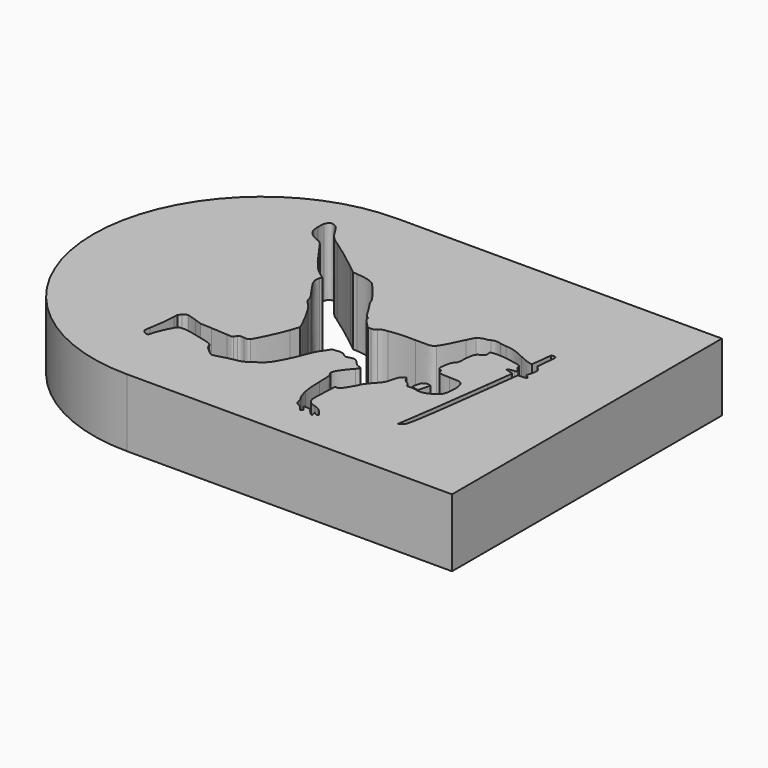
from build123d import *

# Parameters (mm, degrees)
F1_DEPTH = 5.842
F3_DEPTH = 25.4


# Not quite as in the source:
# - ends of sketch curves that miss each other by under 0.0002 mm in the source are joined


with BuildPart() as f1:
    # F0 (on Top) → F1 (new body)
    with BuildSketch(Plane.XY):
        with BuildLine():
            ThreePointArc((0, 14.5415), (-14.5415, 0), (0, -14.5415))
            Line((0, -14.5415), (28.0035, -14.5415))
            Line((28.0035, -14.5415), (28.0035, 14.5415))
            Line((28.0035, 14.5415), (0, 14.5415))
        make_face()
    extrude(amount=-F1_DEPTH)

    # F2 (on face) → F3 (cut)
    with BuildSketch(Plane.XY):
        with BuildLine():
            add(Edge.make_bspline(
                [(-3.3505654062, 10.8393135056), (-3.2275024062, 11.2703769056), (-2.9634440062, 11.3611057056), (-2.5826726062, 11.1031687056)],
                knots=[0, 0, 0, 0, 1, 1, 1, 1], degree=3))
            add(Edge.make_bspline(
                [(-3.3873192062, 10.2314661056), (-3.3936946062, 10.4726137056), (-3.3771592062, 10.7461463056), (-3.3505654062, 10.8393135056)],
                knots=[0, 0, 0, 0, 1, 1, 1, 1], degree=3))
            add(Edge.make_bspline(
                [(-2.8288748062, 9.0599165056), (-3.2257752062, 9.3249655056), (-3.3713934062, 9.6304513056), (-3.3873192062, 10.2314661056)],
                knots=[0, 0, 0, 0, 1, 1, 1, 1], degree=3))
            add(Edge.make_bspline(
                [(-2.3834096062, 8.8114283056), (-2.4746972062, 8.8454389056), (-2.6751540062, 8.9572751056), (-2.8288748062, 9.0599165056)],
                knots=[0, 0, 0, 0, 1, 1, 1, 1], degree=3))
            add(Edge.make_bspline(
                [(-1.0314946062, 7.4019823056), (-1.8672816062, 8.6240525056), (-1.8597632062, 8.6162039056), (-2.3834096062, 8.8114283056)],
                knots=[0, 0, 0, 0, 1, 1, 1, 1], degree=3))
            add(Edge.make_bspline(
                [(1.0526515938, 4.9585023056), (0.4475473938, 5.3825299056), (-0.0464826062, 5.9617261056), (-1.0314946062, 7.4019823056)],
                knots=[0, 0, 0, 0, 1, 1, 1, 1], degree=3))
            Line((1.0526515938, 4.9585023056), (1.4337023938, 4.6914975056))
            Line((1.4337023938, 4.6914975056), (1.3601947938, 4.4854019056))
            add(Edge.make_bspline(
                [(1.9874985938, 2.8520803056), (1.3599407938, 3.6886801056), (1.2126969938, 4.0720423056), (1.3601947938, 4.4854019056)],
                knots=[0, 0, 0, 0, 1, 1, 1, 1], degree=3))
            add(Edge.make_bspline(
                [(2.6965141938, 1.6528701056), (2.6965141938, 1.8108835056), (2.4284933938, 2.2641973056), (1.9874985938, 2.8520803056)],
                knots=[0, 0, 0, 0, 1, 1, 1, 1], degree=3))
            add(Edge.make_bspline(
                [(3.1149791938, 1.0430923056), (2.9105853938, 1.2135517056), (2.6965141938, 1.5254891056), (2.6965141938, 1.6528701056)],
                knots=[0, 0, 0, 0, 1, 1, 1, 1], degree=3))
            add(Edge.make_bspline(
                [(3.4769545938, 0.6155341056), (3.3687251938, 0.7749191056), (3.2058349938, 0.9673241056), (3.1149791938, 1.0430923056)],
                knots=[0, 0, 0, 0, 1, 1, 1, 1], degree=3))
            add(Edge.make_bspline(
                [(4.6368709938, -1.5235268944), (4.4779685938, -1.1114626944), (3.7972231938, 0.1439069056), (3.4769545938, 0.6155341056)],
                knots=[0, 0, 0, 0, 1, 1, 1, 1], degree=3))
            Line((4.6368709938, -1.5235268944), (4.7843433938, -1.9058984944))
            Line((4.7843433938, -1.9058984944), (4.5295305938, -2.6590846944))
            add(Edge.make_bspline(
                [(3.2766247938, -5.3463792944), (3.5066725938, -5.0567938944), (4.2781721938, -3.4020600944), (4.5295305938, -2.6590846944)],
                knots=[0, 0, 0, 0, 1, 1, 1, 1], degree=3))
            add(Edge.make_bspline(
                [(2.8130493938, -5.4498080944), (3.1617659938, -5.4824724944), (3.1699701938, -5.4806436944), (3.2766247938, -5.3463792944)],
                knots=[0, 0, 0, 0, 1, 1, 1, 1], degree=3))
            add(Edge.make_bspline(
                [(2.3198829938, -5.5551926944), (2.4545029938, -5.4200900944), (2.4671521938, -5.4173976944), (2.8130493938, -5.4498080944)],
                knots=[0, 0, 0, 0, 1, 1, 1, 1], degree=3))
            add(Edge.make_bspline(
                [(2.1355297938, -5.7769092944), (2.1609297938, -5.7312146944), (2.2438861938, -5.6314434944), (2.3198829938, -5.5551926944)],
                knots=[0, 0, 0, 0, 1, 1, 1, 1], degree=3))
            add(Edge.make_bspline(
                [(1.6304253938, -5.8127232944), (2.0435309938, -5.8552428944), (2.0939753938, -5.8516614944), (2.1355297938, -5.7769092944)],
                knots=[0, 0, 0, 0, 1, 1, 1, 1], degree=3))
            add(Edge.make_bspline(
                [(0.2032247938, -5.7259568944), (0.7357865938, -5.7476992944), (1.3780255938, -5.7867136944), (1.6304253938, -5.8127232944)],
                knots=[0, 0, 0, 0, 1, 1, 1, 1], degree=3))
            Line((0.2032247938, -5.7259568944), (-0.7650486062, -5.6864598944))
            Line((-0.7650486062, -5.6864598944), (-1.3459974062, -5.4790942944))
            add(Edge.make_bspline(
                [(-2.1341086062, -5.2478526944), (-2.0201642062, -5.2609844944), (-1.6655294062, -5.3650482944), (-1.3459974062, -5.4790942944)],
                knots=[0, 0, 0, 0, 1, 1, 1, 1], degree=3))
            add(Edge.make_bspline(
                [(-2.5577298062, -5.4404354944), (-2.3551648062, -5.2378704944), (-2.3279106062, -5.2254752944), (-2.1341086062, -5.2478526944)],
                knots=[0, 0, 0, 0, 1, 1, 1, 1], degree=3))
            Line((-2.5577298062, -5.4404354944), (-2.7741886062, -5.6568942944))
            Line((-2.7741886062, -5.6568942944), (-2.7741886062, -6.0245084944))
            add(Edge.make_bspline(
                [(-3.0388058062, -8.2597592944), (-2.9170128062, -7.6244290944), (-2.7741886062, -6.4181576944), (-2.7741886062, -6.0245084944)],
                knots=[0, 0, 0, 0, 1, 1, 1, 1], degree=3))
            add(Edge.make_bspline(
                [(-2.9799540062, -8.9563288944), (-3.1350210062, -8.7916860944), (-3.1367990062, -8.7707818944), (-3.0388058062, -8.2597592944)],
                knots=[0, 0, 0, 0, 1, 1, 1, 1], degree=3))
            add(Edge.make_bspline(
                [(-2.5392640062, -9.1113958944), (-2.6438866062, -9.1760642944), (-2.8369520062, -9.1081446944), (-2.9799540062, -8.9563288944)],
                knots=[0, 0, 0, 0, 1, 1, 1, 1], degree=3))
            add(Edge.make_bspline(
                [(-2.4057108062, -8.7382190944), (-2.4435822062, -8.9214800944), (-2.5037040062, -9.0894248944), (-2.5392640062, -9.1113958944)],
                knots=[0, 0, 0, 0, 1, 1, 1, 1], degree=3))
            add(Edge.make_bspline(
                [(-1.6354304062, -7.0924006944), (-1.8189708062, -7.2759156944), (-2.3284694062, -8.3645342944), (-2.4057108062, -8.7382190944)],
                knots=[0, 0, 0, 0, 1, 1, 1, 1], degree=3))
            add(Edge.make_bspline(
                [(-1.2150604062, -6.9773132944), (-1.4721846062, -6.9768306944), (-1.5379198062, -6.9948900944), (-1.6354304062, -7.0924006944)],
                knots=[0, 0, 0, 0, 1, 1, 1, 1], degree=3))
            add(Edge.make_bspline(
                [(0.8847829938, -7.3951940944), (-0.0074682062, -7.1444198944), (-0.8440934062, -6.9779228944), (-1.2150604062, -6.9773132944)],
                knots=[0, 0, 0, 0, 1, 1, 1, 1], degree=3))
            add(Edge.make_bspline(
                [(1.6190461938, -7.7483556944), (1.5512535938, -7.5863544944), (1.5318733938, -7.5770326944), (0.8847829938, -7.3951940944)],
                knots=[0, 0, 0, 0, 1, 1, 1, 1], degree=3))
            add(Edge.make_bspline(
                [(1.8173947938, -8.0838388944), (1.7466049938, -7.9908240944), (1.6573493938, -7.8398464944), (1.6190461938, -7.7483556944)],
                knots=[0, 0, 0, 0, 1, 1, 1, 1], degree=3))
            add(Edge.make_bspline(
                [(2.6697171938, -8.7680894944), (2.5522929938, -8.7680894944), (2.0018495938, -8.3261802944), (1.8173947938, -8.0838388944)],
                knots=[0, 0, 0, 0, 1, 1, 1, 1], degree=3))
            add(Edge.make_bspline(
                [(3.4470079938, -8.5743636944), (3.0742629938, -8.6809166944), (2.7244795938, -8.7680894944), (2.6697171938, -8.7680894944)],
                knots=[0, 0, 0, 0, 1, 1, 1, 1], degree=3))
            add(Edge.make_bspline(
                [(4.4755301938, -8.3370006944), (4.2825663938, -8.3610036944), (3.8197529938, -8.4678106944), (3.4470079938, -8.5743636944)],
                knots=[0, 0, 0, 0, 1, 1, 1, 1], degree=3))
            add(Edge.make_bspline(
                [(5.7562235938, -7.6816552944), (4.9934869938, -8.2261550944), (4.8735227938, -8.2875214944), (4.4755301938, -8.3370006944)],
                knots=[0, 0, 0, 0, 1, 1, 1, 1], degree=3))
            add(Edge.make_bspline(
                [(6.4918837938, -6.9844506944), (6.3146425938, -7.2510744944), (6.1780667938, -7.3805128944), (5.7562235938, -7.6816552944)],
                knots=[0, 0, 0, 0, 1, 1, 1, 1], degree=3))
            add(Edge.make_bspline(
                [(7.4134719938, -5.1370832944), (7.1996801938, -5.7229342944), (6.8062849938, -6.5115534944), (6.4918837938, -6.9844506944)],
                knots=[0, 0, 0, 0, 1, 1, 1, 1], degree=3))
            add(Edge.make_bspline(
                [(8.0773009938, -3.7124480944), (7.9343497938, -3.8755160944), (7.6553561938, -4.4742702944), (7.4134719938, -5.1370832944)],
                knots=[0, 0, 0, 0, 1, 1, 1, 1], degree=3))
            add(Edge.make_bspline(
                [(8.3400131938, -3.3308892944), (8.2583013938, -3.4691414944), (8.1400897938, -3.6408454944), (8.0773009938, -3.7124480944)],
                knots=[0, 0, 0, 0, 1, 1, 1, 1], degree=3))
            add(Edge.make_bspline(
                [(8.6434923938, -3.0716060944), (8.5114377938, -3.0783624944), (8.4666321938, -3.1166148944), (8.3400131938, -3.3308892944)],
                knots=[0, 0, 0, 0, 1, 1, 1, 1], degree=3))
            add(Edge.make_bspline(
                [(8.9918025938, -3.0366302944), (8.8854527938, -3.0514892944), (8.7287093938, -3.0672372944), (8.6434923938, -3.0716060944)],
                knots=[0, 0, 0, 0, 1, 1, 1, 1], degree=3))
            add(Edge.make_bspline(
                [(9.6258627938, -3.2060990944), (9.4464371938, -3.0459012944), (9.2674433938, -2.9980730944), (8.9918025938, -3.0366302944)],
                knots=[0, 0, 0, 0, 1, 1, 1, 1], degree=3))
            add(Edge.make_bspline(
                [(10.2087927938, -3.2670082944), (9.8359461938, -3.3716308944), (9.8079807938, -3.3686844944), (9.6258627938, -3.2060990944)],
                knots=[0, 0, 0, 0, 1, 1, 1, 1], degree=3))
            add(Edge.make_bspline(
                [(11.0254027938, -3.5898930944), (10.7011463938, -3.2156240944), (10.5728001938, -3.1648748944), (10.2087927938, -3.2670082944)],
                knots=[0, 0, 0, 0, 1, 1, 1, 1], degree=3))
            add(Edge.make_bspline(
                [(11.4640099938, -3.9033290944), (11.3044725938, -3.8763796944), (11.2233957938, -3.8184422944), (11.0254027938, -3.5898930944)],
                knots=[0, 0, 0, 0, 1, 1, 1, 1], degree=3))
            add(Edge.make_bspline(
                [(11.6861837938, -4.0052846944), (11.6716549938, -3.9674132944), (11.5716805938, -3.9215154944), (11.4640099938, -3.9033290944)],
                knots=[0, 0, 0, 0, 1, 1, 1, 1], degree=3))
            add(Edge.make_bspline(
                [(11.5012717938, -4.3054872944), (11.6230139938, -4.1722642944), (11.7014237938, -4.0449848944), (11.6861837938, -4.0052846944)],
                knots=[0, 0, 0, 0, 1, 1, 1, 1], degree=3))
            add(Edge.make_bspline(
                [(10.5397801938, -5.7960100944), (10.5412533938, -5.5009890944), (10.8591089938, -5.0082290944), (11.5012717938, -4.3054872944)],
                knots=[0, 0, 0, 0, 1, 1, 1, 1], degree=3))
            add(Edge.make_bspline(
                [(10.6534959938, -6.0177774944), (10.5908087938, -5.9253722944), (10.5396277938, -5.8256010944), (10.5397801938, -5.7960100944)],
                knots=[0, 0, 0, 0, 1, 1, 1, 1], degree=3))
            add(Edge.make_bspline(
                [(10.7944913938, -7.3195782944), (10.7685833938, -6.2311374944), (10.7629445938, -6.1790420944), (10.6534959938, -6.0177774944)],
                knots=[0, 0, 0, 0, 1, 1, 1, 1], degree=3))
            add(Edge.make_bspline(
                [(10.9251997938, -8.9564812944), (10.8437673938, -8.5615874944), (10.8156749938, -8.2095942944), (10.7944913938, -7.3195782944)],
                knots=[0, 0, 0, 0, 1, 1, 1, 1], degree=3))
            add(Edge.make_bspline(
                [(11.3379243938, -10.0268626944), (11.1851433938, -9.8455066944), (11.0204243938, -9.4182786944), (10.9251997938, -8.9564812944)],
                knots=[0, 0, 0, 0, 1, 1, 1, 1], degree=3))
            add(Edge.make_bspline(
                [(11.4311169938, -10.3223408944), (11.4135147938, -10.1997604944), (11.3715539938, -10.0667914944), (11.3379243938, -10.0268626944)],
                knots=[0, 0, 0, 0, 1, 1, 1, 1], degree=3))
            add(Edge.make_bspline(
                [(11.8227087938, -10.8226446944), (11.5826025938, -10.7223400944), (11.4674643938, -10.5752486944), (11.4311169938, -10.3223408944)],
                knots=[0, 0, 0, 0, 1, 1, 1, 1], degree=3))
            add(Edge.make_bspline(
                [(12.1231907938, -11.0862966944), (12.0489465938, -10.9793118944), (11.9137169938, -10.8606938944), (11.8227087938, -10.8226446944)],
                knots=[0, 0, 0, 0, 1, 1, 1, 1], degree=3))
            add(Edge.make_bspline(
                [(12.4579627938, -11.2805050944), (12.3635509938, -11.3588640944), (12.2779021938, -11.3092070944), (12.1231907938, -11.0862966944)],
                knots=[0, 0, 0, 0, 1, 1, 1, 1], degree=3))
            add(Edge.make_bspline(
                [(12.3512319938, -10.9554104944), (12.5451863938, -11.1820038944), (12.5519173938, -11.2025270944), (12.4579627938, -11.2805050944)],
                knots=[0, 0, 0, 0, 1, 1, 1, 1], degree=3))
            Line((12.3512319938, -10.9554104944), (12.1780039938, -10.7530486944))
            Line((12.1780039938, -10.7530486944), (12.4270255938, -10.7530486944))
            add(Edge.make_bspline(
                [(12.9128767938, -10.9738508944), (12.8514849938, -10.8123576944), (12.7209543938, -10.7530486944), (12.4270255938, -10.7530486944)],
                knots=[0, 0, 0, 0, 1, 1, 1, 1], degree=3))
            add(Edge.make_bspline(
                [(13.0289547938, -11.0919354944), (12.9898133938, -11.0919354944), (12.9375655938, -11.0387986944), (12.9128767938, -10.9738508944)],
                knots=[0, 0, 0, 0, 1, 1, 1, 1], degree=3))
            add(Edge.make_bspline(
                [(13.1637271938, -11.2250822944), (13.1287513938, -11.1518540944), (13.0680961938, -11.0919354944), (13.0289547938, -11.0919354944)],
                knots=[0, 0, 0, 0, 1, 1, 1, 1], degree=3))
            add(Edge.make_bspline(
                [(13.4267187938, -11.3095626944), (13.4825225938, -11.4550284944), (13.2357107938, -11.3757296944), (13.1637271938, -11.2250822944)],
                knots=[0, 0, 0, 0, 1, 1, 1, 1], degree=3))
            add(Edge.make_bspline(
                [(13.3651999938, -11.0995554944), (13.3818369938, -11.1702944944), (13.4095229938, -11.2648078944), (13.4267187938, -11.3095626944)],
                knots=[0, 0, 0, 0, 1, 1, 1, 1], degree=3))
            Line((13.3651999938, -11.0995554944), (13.3348977938, -10.9709044944))
            Line((13.3348977938, -10.9709044944), (13.4399013938, -11.0798450944))
            add(Edge.make_bspline(
                [(13.7656817938, -11.1161162944), (13.8107159938, -11.2334642944), (13.5611863938, -11.2056766944), (13.4399013938, -11.0798450944)],
                knots=[0, 0, 0, 0, 1, 1, 1, 1], degree=3))
            add(Edge.make_bspline(
                [(13.2264397938, -10.4739026944), (13.4143489938, -10.6175650944), (13.7090397938, -10.9685422944), (13.7656817938, -11.1161162944)],
                knots=[0, 0, 0, 0, 1, 1, 1, 1], degree=3))
            add(Edge.make_bspline(
                [(12.7633723938, -10.2558944944), (12.9115559938, -10.2943754944), (13.1199375938, -10.3924702944), (13.2264397938, -10.4739026944)],
                knots=[0, 0, 0, 0, 1, 1, 1, 1], degree=3))
            add(Edge.make_bspline(
                [(12.0906279938, -9.8329336944), (12.2213871938, -10.0686202944), (12.3476251938, -10.1479698944), (12.7633723938, -10.2558944944)],
                knots=[0, 0, 0, 0, 1, 1, 1, 1], degree=3))
            add(Edge.make_bspline(
                [(12.0199905938, -8.0903158944), (11.9475751938, -9.4684690944), (11.9522487938, -9.5834802944), (12.0906279938, -9.8329336944)],
                knots=[0, 0, 0, 0, 1, 1, 1, 1], degree=3))
            Line((12.0199905938, -8.0903158944), (12.0645167938, -7.2430734944))
            Line((12.0645167938, -7.2430734944), (12.2447551938, -7.2281382944))
            add(Edge.make_bspline(
                [(12.5261109938, -7.0829010944), (12.4546353938, -7.1749760944), (12.3720853938, -7.2175972944), (12.2447551938, -7.2281382944)],
                knots=[0, 0, 0, 0, 1, 1, 1, 1], degree=3))
            add(Edge.make_bspline(
                [(13.1625333938, -6.0085572944), (13.1052055938, -6.1597126944), (12.6621025938, -6.9077426944), (12.5261109938, -7.0829010944)],
                knots=[0, 0, 0, 0, 1, 1, 1, 1], degree=3))
            add(Edge.make_bspline(
                [(13.8604237938, -5.0402838944), (13.5216131938, -5.3899402944), (13.2589009938, -5.7544302944), (13.1625333938, -6.0085572944)],
                knots=[0, 0, 0, 0, 1, 1, 1, 1], degree=3))
            add(Edge.make_bspline(
                [(14.4640547938, -3.8166642944), (14.3186397938, -4.4798836944), (14.2306795938, -4.6581916944), (13.8604237938, -5.0402838944)],
                knots=[0, 0, 0, 0, 1, 1, 1, 1], degree=3))
            add(Edge.make_bspline(
                [(14.7380445938, -3.3410492944), (14.5629115938, -3.5024916944), (14.5145245938, -3.5864894944), (14.4640547938, -3.8166642944)],
                knots=[0, 0, 0, 0, 1, 1, 1, 1], degree=3))
            add(Edge.make_bspline(
                [(15.0205687938, -3.2028986944), (14.9639267938, -3.1559086944), (14.9106121938, -3.1819690944), (14.7380445938, -3.3410492944)],
                knots=[0, 0, 0, 0, 1, 1, 1, 1], degree=3))
            add(Edge.make_bspline(
                [(15.0903679938, -3.3467134944), (15.0903679938, -3.2994948944), (15.0589481938, -3.2347756944), (15.0205687938, -3.2028986944)],
                knots=[0, 0, 0, 0, 1, 1, 1, 1], degree=3))
            add(Edge.make_bspline(
                [(15.5182309938, -3.7548406944), (15.3689043938, -3.7074442944), (15.0903679938, -3.4417602944), (15.0903679938, -3.3467134944)],
                knots=[0, 0, 0, 0, 1, 1, 1, 1], degree=3))
            add(Edge.make_bspline(
                [(15.6937449938, -3.9540528944), (15.6496505938, -3.8611142944), (15.5706565938, -3.7714776944), (15.5182309938, -3.7548406944)],
                knots=[0, 0, 0, 0, 1, 1, 1, 1], degree=3))
            add(Edge.make_bspline(
                [(16.0009833938, -4.0939052944), (15.7787333938, -4.1223786944), (15.7722055938, -4.1194068944), (15.6937449938, -3.9540528944)],
                knots=[0, 0, 0, 0, 1, 1, 1, 1], degree=3))
            add(Edge.make_bspline(
                [(16.5166287938, -4.1410222944), (16.3357553938, -4.0932448944), (16.1433249938, -4.0756680944), (16.0009833938, -4.0939052944)],
                knots=[0, 0, 0, 0, 1, 1, 1, 1], degree=3))
            add(Edge.make_bspline(
                [(17.4719227938, -4.1167652944), (17.1669449938, -4.2369834944), (16.9049947938, -4.2436382944), (16.5166287938, -4.1410222944)],
                knots=[0, 0, 0, 0, 1, 1, 1, 1], degree=3))
            add(Edge.make_bspline(
                [(18.3957715938, -3.4327940944), (18.3063127938, -3.6234972944), (17.8314343938, -3.9750586944), (17.4719227938, -4.1167652944)],
                knots=[0, 0, 0, 0, 1, 1, 1, 1], degree=3))
            add(Edge.make_bspline(
                [(18.5272673938, -2.0712016944), (18.5881511938, -2.4226868944), (18.5151769938, -3.1782606944), (18.3957715938, -3.4327940944)],
                knots=[0, 0, 0, 0, 1, 1, 1, 1], degree=3))
            add(Edge.make_bspline(
                [(17.2386745938, -1.3329252944), (18.3122055938, -1.3384116944), (18.4100463938, -1.3944694944), (18.5272673938, -2.0712016944)],
                knots=[0, 0, 0, 0, 1, 1, 1, 1], degree=3))
            add(Edge.make_bspline(
                [(16.1944805938, -1.0538554944), (16.2170103938, -1.2854018944), (16.3783765938, -1.3285310944), (17.2386745938, -1.3329252944)],
                knots=[0, 0, 0, 0, 1, 1, 1, 1], degree=3))
            add(Edge.make_bspline(
                [(16.0527231938, -0.8410796944), (16.1431725938, -0.8842088944), (16.1839141938, -0.9453974944), (16.1944805938, -1.0538554944)],
                knots=[0, 0, 0, 0, 1, 1, 1, 1], degree=3))
            add(Edge.make_bspline(
                [(15.8627565938, -0.2858864944), (15.8029903938, -0.6743286944), (15.8224975938, -0.7313008944), (16.0527231938, -0.8410796944)],
                knots=[0, 0, 0, 0, 1, 1, 1, 1], degree=3))
            add(Edge.make_bspline(
                [(16.1682931938, 0.6071267056), (16.0011357938, 0.4167283056), (15.9461701938, 0.2560225056), (15.8627565938, -0.2858864944)],
                knots=[0, 0, 0, 0, 1, 1, 1, 1], degree=3))
            add(Edge.make_bspline(
                [(16.3486839938, 1.3932059056), (16.3227251938, 0.7919879056), (16.3199311938, 0.7797959056), (16.1682931938, 0.6071267056)],
                knots=[0, 0, 0, 0, 1, 1, 1, 1], degree=3))
            add(Edge.make_bspline(
                [(16.7442127938, 2.5041003056), (16.4755569938, 2.3565263056), (16.3785035938, 2.0839335056), (16.3486839938, 1.3932059056)],
                knots=[0, 0, 0, 0, 1, 1, 1, 1], degree=3))
            add(Edge.make_bspline(
                [(17.0992285938, 2.9984605056), (17.1337725938, 2.7473053056), (17.0991015938, 2.6990199056), (16.7442127938, 2.5041003056)],
                knots=[0, 0, 0, 0, 1, 1, 1, 1], degree=3))
            Line((17.0992285938, 2.9984605056), (17.0674023938, 3.2298545056))
            Line((17.0674023938, 3.2298545056), (17.3890425938, 3.2642969056))
            add(Edge.make_bspline(
                [(18.9392299938, 3.1356967056), (18.2177429938, 3.2684117056), (17.7724047938, 3.3053687056), (17.3890425938, 3.2642969056)],
                knots=[0, 0, 0, 0, 1, 1, 1, 1], degree=3))
            add(Edge.make_bspline(
                [(19.8777091938, 2.7538585056), (19.8109833938, 2.9765149056), (19.8163681938, 2.9743305056), (18.9392299938, 3.1356967056)],
                knots=[0, 0, 0, 0, 1, 1, 1, 1], degree=3))
            add(Edge.make_bspline(
                [(20.0791311938, 2.3960995056), (20.0004419938, 2.4857107056), (19.9098147938, 2.6466959056), (19.8777091938, 2.7538585056)],
                knots=[0, 0, 0, 0, 1, 1, 1, 1], degree=3))
            add(Edge.make_bspline(
                [(20.0406247938, 2.1246243056), (20.2599537938, 2.1249545056), (20.2679039938, 2.1810885056), (20.0791311938, 2.3960995056)],
                knots=[0, 0, 0, 0, 1, 1, 1, 1], degree=3))
            add(Edge.make_bspline(
                [(19.4959979938, 1.9811397056), (19.4959979938, 2.0391533056), (19.8192129938, 2.1242941056), (20.0406247938, 2.1246243056)],
                knots=[0, 0, 0, 0, 1, 1, 1, 1], degree=3))
            add(Edge.make_bspline(
                [(19.9959969938, 1.8113915056), (19.7177907938, 1.8582037056), (19.4959979938, 1.9335147056), (19.4959979938, 1.9811397056)],
                knots=[0, 0, 0, 0, 1, 1, 1, 1], degree=3))
            add(Edge.make_bspline(
                [(20.1535023938, 1.6015621056), (20.1808581938, 1.7774063056), (20.1783943938, 1.7807083056), (19.9959969938, 1.8113915056)],
                knots=[0, 0, 0, 0, 1, 1, 1, 1], degree=3))
            add(Edge.make_bspline(
                [(19.8809095938, -0.5378290944), (20.0155549938, 0.5405787056), (20.1382115938, 1.5032895056), (20.1535023938, 1.6015621056)],
                knots=[0, 0, 0, 0, 1, 1, 1, 1], degree=3))
            add(Edge.make_bspline(
                [(18.7495427938, -8.7318690944), (18.8561211938, -8.2594798944), (19.4904861938, -3.6651024944), (19.8809095938, -0.5378290944)],
                knots=[0, 0, 0, 0, 1, 1, 1, 1], degree=3))
            add(Edge.make_bspline(
                [(18.9989199938, -8.6381176944), (18.7602361938, -8.8145968944), (18.7281559938, -8.8266618944), (18.7495427938, -8.7318690944)],
                knots=[0, 0, 0, 0, 1, 1, 1, 1], degree=3))
            add(Edge.make_bspline(
                [(19.2281549938, -8.2700462944), (19.1763135938, -8.4499798944), (19.1105529938, -8.5555676944), (18.9989199938, -8.6381176944)],
                knots=[0, 0, 0, 0, 1, 1, 1, 1], degree=3))
            add(Edge.make_bspline(
                [(20.2715869938, -1.0703908944), (19.8048365938, -4.8771904944), (19.3990969938, -7.6768038944), (19.2281549938, -8.2700462944)],
                knots=[0, 0, 0, 0, 1, 1, 1, 1], degree=3))
            add(Edge.make_bspline(
                [(20.5965799938, 1.5197233056), (20.5761837938, 1.3866019056), (20.4299305938, 0.2210467056), (20.2715869938, -1.0703908944)],
                knots=[0, 0, 0, 0, 1, 1, 1, 1], degree=3))
            Line((20.5965799938, 1.5197233056), (20.6336893938, 1.7618107056))
            Line((20.6336893938, 1.7618107056), (20.9483953938, 1.7860169056))
            add(Edge.make_bspline(
                [(21.3071449938, 1.9844671056), (21.4210385938, 1.8586355056), (21.3448893938, 1.8164969056), (20.9483953938, 1.7860169056)],
                knots=[0, 0, 0, 0, 1, 1, 1, 1], degree=3))
            add(Edge.make_bspline(
                [(21.1616029938, 2.0764913056), (21.1958421938, 2.0764913056), (21.2613487938, 2.0350893056), (21.3071449938, 1.9844671056)],
                knots=[0, 0, 0, 0, 1, 1, 1, 1], degree=3))
            add(Edge.make_bspline(
                [(21.1414861938, 2.4460613056), (21.0450677938, 2.1578729056), (21.0494873938, 2.0764913056), (21.1616029938, 2.0764913056)],
                knots=[0, 0, 0, 0, 1, 1, 1, 1], degree=3))
            add(Edge.make_bspline(
                [(21.2376759938, 2.9657199056), (21.2370409938, 2.8361291056), (21.1937339938, 2.6022713056), (21.1414861938, 2.4460613056)],
                knots=[0, 0, 0, 0, 1, 1, 1, 1], degree=3))
            add(Edge.make_bspline(
                [(21.0402163938, 3.4000345056), (21.2190069938, 3.2212693056), (21.2387427938, 3.1778099056), (21.2376759938, 2.9657199056)],
                knots=[0, 0, 0, 0, 1, 1, 1, 1], degree=3))
            Line((21.0402163938, 3.4000345056), (20.8415629938, 3.5987133056))
            Line((20.8415629938, 3.5987133056), (20.9271863938, 4.4521025056))
            add(Edge.make_bspline(
                [(20.9821265938, 5.3854509056), (20.9989921938, 5.3414581056), (20.9742779938, 4.9214437056), (20.9271863938, 4.4521025056)],
                knots=[0, 0, 0, 0, 1, 1, 1, 1], degree=3))
            add(Edge.make_bspline(
                [(20.5589879938, 5.4049073056), (20.5623153938, 5.5011987056), (20.9444329938, 5.4836473056), (20.9821265938, 5.3854509056)],
                knots=[0, 0, 0, 0, 1, 1, 1, 1], degree=3))
            add(Edge.make_bspline(
                [(20.3552545938, 3.6458303056), (20.3779367938, 3.6684871056), (20.5503773938, 5.1575367056), (20.5589879938, 5.4049073056)],
                knots=[0, 0, 0, 0, 1, 1, 1, 1], degree=3))
            add(Edge.make_bspline(
                [(19.1252595938, 4.0586057056), (19.7361549938, 3.7568283056), (20.2828137938, 3.5733895056), (20.3552545938, 3.6458303056)],
                knots=[0, 0, 0, 0, 1, 1, 1, 1], degree=3))
            add(Edge.make_bspline(
                [(17.3686717938, 4.5945711056), (17.8184041938, 4.5936059056), (18.4037471938, 4.4149931056), (19.1252595938, 4.0586057056)],
                knots=[0, 0, 0, 0, 1, 1, 1, 1], degree=3))
            add(Edge.make_bspline(
                [(16.8332397938, 4.6666055056), (16.9796961938, 4.6273117056), (17.2206405938, 4.5948759056), (17.3686717938, 4.5945711056)],
                knots=[0, 0, 0, 0, 1, 1, 1, 1], degree=3))
            add(Edge.make_bspline(
                [(16.0228527938, 4.6423993056), (16.2370001938, 4.7571565056), (16.4699435938, 4.7641161056), (16.8332397938, 4.6666055056)],
                knots=[0, 0, 0, 0, 1, 1, 1, 1], degree=3))
            add(Edge.make_bspline(
                [(15.7413445938, 4.5455745056), (15.7968181938, 4.5455745056), (15.9235133938, 4.5891609056), (16.0228527938, 4.6423993056)],
                knots=[0, 0, 0, 0, 1, 1, 1, 1], degree=3))
            add(Edge.make_bspline(
                [(15.0342339938, 4.2683335056), (15.1544013938, 4.3975941056), (15.5318453938, 4.5455745056), (15.7413445938, 4.5455745056)],
                knots=[0, 0, 0, 0, 1, 1, 1, 1], degree=3))
            add(Edge.make_bspline(
                [(14.6797769938, 3.6257135056), (14.8060657938, 3.9053167056), (14.9655777938, 4.1944957056), (15.0342339938, 4.2683335056)],
                knots=[0, 0, 0, 0, 1, 1, 1, 1], degree=3))
            add(Edge.make_bspline(
                [(13.6749275938, 1.7227709056), (13.8424913938, 1.9181985056), (14.2989039938, 2.7825605056), (14.6797769938, 3.6257135056)],
                knots=[0, 0, 0, 0, 1, 1, 1, 1], degree=3))
            add(Edge.make_bspline(
                [(12.0403105938, 1.4744351056), (13.3081769938, 1.4404245056), (13.4515091938, 1.4621923056), (13.6749275938, 1.7227709056)],
                knots=[0, 0, 0, 0, 1, 1, 1, 1], degree=3))
            add(Edge.make_bspline(
                [(9.7890831938, 1.3514229056), (10.7314993938, 1.4874653056), (11.0025427938, 1.5022735056), (12.0403105938, 1.4744351056)],
                knots=[0, 0, 0, 0, 1, 1, 1, 1], degree=3))
            add(Edge.make_bspline(
                [(9.0654371938, 1.0833259056), (9.2479615938, 1.2658503056), (9.2808799938, 1.2780423056), (9.7890831938, 1.3514229056)],
                knots=[0, 0, 0, 0, 1, 1, 1, 1], degree=3))
            add(Edge.make_bspline(
                [(8.6398093938, 0.9145683056), (8.8686125938, 0.9145683056), (8.9150945938, 0.9330087056), (9.0654371938, 1.0833259056)],
                knots=[0, 0, 0, 0, 1, 1, 1, 1], degree=3))
            Line((8.6398093938, 0.9145683056), (8.3829645938, 0.9145683056))
            Line((8.3829645938, 0.9145683056), (7.9878675938, 1.3139833056))
            add(Edge.make_bspline(
                [(7.5774289938, 1.8586355056), (7.5886557938, 1.7523365056), (7.6987139938, 1.6062865056), (7.9878675938, 1.3139833056)],
                knots=[0, 0, 0, 0, 1, 1, 1, 1], degree=3))
            add(Edge.make_bspline(
                [(7.4155039938, 2.0746879056), (7.5224125938, 2.0230243056), (7.5662275938, 1.9645789056), (7.5774289938, 1.8586355056)],
                knots=[0, 0, 0, 0, 1, 1, 1, 1], degree=3))
            add(Edge.make_bspline(
                [(6.9910191938, 2.6421493056), (7.1940413938, 2.2793357056), (7.3084175938, 2.1264277056), (7.4155039938, 2.0746879056)],
                knots=[0, 0, 0, 0, 1, 1, 1, 1], degree=3))
            add(Edge.make_bspline(
                [(6.4762627938, 3.4516727056), (6.6065139938, 3.2795623056), (6.8381619938, 2.9153009056), (6.9910191938, 2.6421493056)],
                knots=[0, 0, 0, 0, 1, 1, 1, 1], degree=3))
            add(Edge.make_bspline(
                [(6.1641729938, 4.0219281056), (6.2072259938, 3.8747097056), (6.3408045938, 3.6306411056), (6.4762627938, 3.4516727056)],
                knots=[0, 0, 0, 0, 1, 1, 1, 1], degree=3))
            add(Edge.make_bspline(
                [(5.4283857938, 5.1023425056), (5.9508129938, 4.4513913056), (6.1046607938, 4.2254837056), (6.1641729938, 4.0219281056)],
                knots=[0, 0, 0, 0, 1, 1, 1, 1], degree=3))
            add(Edge.make_bspline(
                [(4.6431193938, 6.0583477056), (4.7117247938, 5.9852211056), (5.0651149938, 5.5549959056), (5.4283857938, 5.1023425056)],
                knots=[0, 0, 0, 0, 1, 1, 1, 1], degree=3))
            add(Edge.make_bspline(
                [(2.9330643938, 6.5501933056), (3.6955215938, 6.5021365056), (4.4232061938, 6.2928405056), (4.6431193938, 6.0583477056)],
                knots=[0, 0, 0, 0, 1, 1, 1, 1], degree=3))
            Line((2.9330643938, 6.5501933056), (2.5853891938, 6.5721135056))
            Line((2.5853891938, 6.5721135056), (1.9268687938, 7.1002303056))
            add(Edge.make_bspline(
                [(-0.8054600062, 9.1349227056), (-0.0911866062, 8.6574789056), (0.9765277938, 7.8623827056), (1.9268687938, 7.1002303056)],
                knots=[0, 0, 0, 0, 1, 1, 1, 1], degree=3))
            add(Edge.make_bspline(
                [(-2.0946624062, 10.4762205056), (-1.7152372062, 9.8135345056), (-1.5257278062, 9.6163797056), (-0.8054600062, 9.1349227056)],
                knots=[0, 0, 0, 0, 1, 1, 1, 1], degree=3))
            add(Edge.make_bspline(
                [(-2.5826726062, 11.1031687056), (-2.4230082062, 10.9950155056), (-2.3045934062, 10.8428949056), (-2.0946624062, 10.4762205056)],
                knots=[0, 0, 0, 0, 1, 1, 1, 1], degree=3))
        make_face()
        with BuildLine():
            add(Edge.make_bspline(
                [(16.1483795938, -3.9169942944), (16.1933629938, -3.9879110944), (16.6773853938, -4.1289318944), (16.7068239938, -4.0797066944)],
                knots=[0, 0, 0, 0, 1, 1, 1, 1], degree=3))
            add(Edge.make_bspline(
                [(16.1126417938, -3.8299484944), (16.1103811938, -3.8432580944), (16.1264593938, -3.8824248944), (16.1483795938, -3.9169942944)],
                knots=[0, 0, 0, 0, 1, 1, 1, 1], degree=3))
            add(Edge.make_bspline(
                [(16.2792657938, -3.1739426944), (16.2174929938, -3.3865152944), (16.1285167938, -3.7367812944), (16.1126417938, -3.8299484944)],
                knots=[0, 0, 0, 0, 1, 1, 1, 1], degree=3))
            Line((16.2792657938, -3.1739426944), (16.6514265938, -2.9892084944))
            add(Edge.make_bspline(
                [(16.9648625938, -3.0739936944), (16.9565059938, -3.0656116944), (16.8154597938, -3.0274608944), (16.6514265938, -2.9892084944)],
                knots=[0, 0, 0, 0, 1, 1, 1, 1], degree=3))
            add(Edge.make_bspline(
                [(16.7068239938, -4.0797066944), (16.7411647938, -4.0223026944), (16.9804581938, -3.0895892944), (16.9648625938, -3.0739936944)],
                knots=[0, 0, 0, 0, 1, 1, 1, 1], degree=3))
        make_face(mode=Mode.SUBTRACT)
    extrude(amount=-F3_DEPTH, mode=Mode.SUBTRACT)


solid = f1.part
